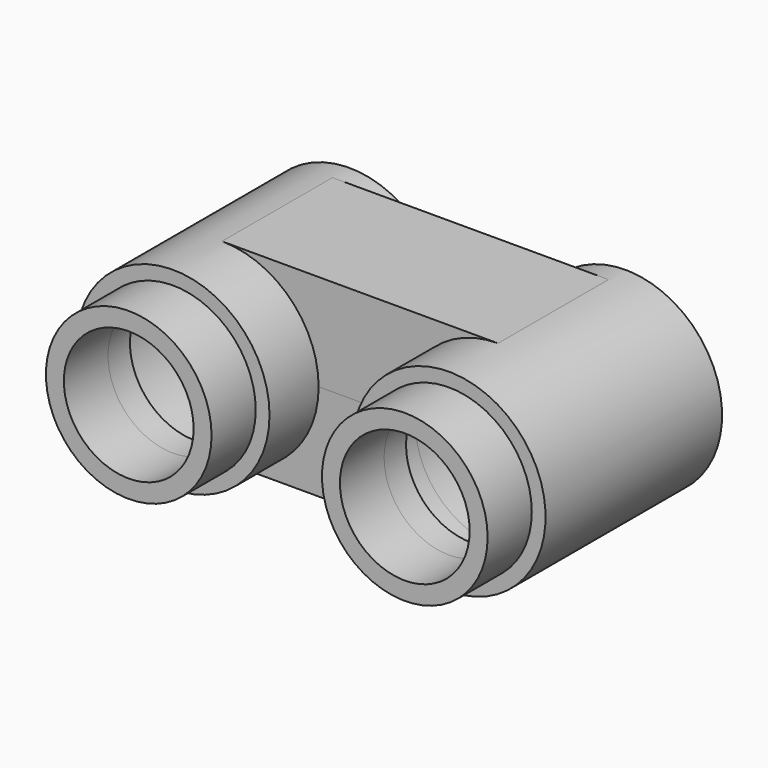
from build123d import *
from build123d import SkipClean  # not in build123d's __all__

# Parameters (mm, degrees)
F1_R           = 8.89
F1_R_2         = 5.969
F3_R           = 7.62
F3_R_2         = 5.969
F4_R           = 7.62
F4_R_2         = 5.969
F5_DEPTH       = 5.08
F6_DEPTH       = 25.4
F6_DEPTH_BACK  = 25.4
F7_R           = 7.62
F8_R           = 7.62
F9_DEPTH       = 17.78
F0_W           = 25.4
F0_H           = 12.7
F10_DEPTH      = 8.89
F10_DEPTH_BACK = 8.89
F11_DEPTH      = 17.78


# Not quite as in the source:
# - a feature of the source that left no trace in its solid (it failed there, or was rolled back) is left out


with BuildPart() as f2:
    # F2: sweep along a path in F0
    with BuildLine(Plane.XY) as f2_path:
        Line((0, 0), (0, 35.9156))
        ThreePointArc((0, 35.9156), (12.7, 48.6156), (25.4, 35.9156))
        Line((25.4, 35.9156), (25.4, 0))
    # F1 (on Front) → F2 (sweep)
    with BuildSketch(Plane.XZ):
        Circle(F1_R)
        Circle(F1_R_2, mode=Mode.SUBTRACT)
    sweep(path=f2_path.line)

    # F3 (on face) + F4 (on face) → F5 (join)
    with BuildSketch(Plane.XZ):
        Circle(F3_R)
        Circle(F3_R_2, mode=Mode.SUBTRACT)
    with BuildSketch(Plane.XZ):
        with Locations((25.4, 0)):
            Circle(F4_R)
        with Locations((25.4, 0)):
            Circle(F4_R_2, mode=Mode.SUBTRACT)
    with SkipClean():  # cleaning this boolean's faces spoils the solid; the shape is the same uncleaned
        extrude(amount=F5_DEPTH)

    # F0 (on Top) → F6 (cut, two sides)
    with BuildSketch(Plane.XY) as f6_sk:
        with BuildLine():
            Line((-12.2957220301, 20.301265642), (0, 20.301265642))
            Line((0, 20.301265642), (0, 35.9156))
            ThreePointArc((0, 35.9156), (3.7197438789, 44.8958561211), (12.7, 48.6156))
            ThreePointArc((12.7, 48.6156), (21.6802561211, 44.8958561211), (25.4, 35.9156))
            Line((25.4, 35.9156), (25.4, 20.301265642))
            Line((25.4, 20.301265642), (40.2239970863, 20.301265642))
            Line((40.2239970863, 20.301265642), (40.2239970863, 60.9702691436))
            Line((40.2239970863, 60.9702691436), (-12.2957220301, 60.9702691436))
            Line((-12.2957220301, 60.9702691436), (-12.2957220301, 20.301265642))
        make_face()
        with BuildLine():
            Line((0, 35.9156), (0, 20.301265642))
            Line((0, 20.301265642), (12.7, 20.301265642))
            Line((12.7, 20.301265642), (12.7, 48.6156))
            ThreePointArc((12.7, 48.6156), (3.7197438789, 44.8958561211), (0, 35.9156))
        make_face()
        with BuildLine():
            Line((12.7, 20.301265642), (25.4, 20.301265642))
            Line((25.4, 20.301265642), (25.4, 35.9156))
            ThreePointArc((25.4, 35.9156), (21.6802561211, 44.8958561211), (12.7, 48.6156))
            Line((12.7, 48.6156), (12.7, 20.301265642))
        make_face()
    extrude(amount=-F6_DEPTH, mode=Mode.SUBTRACT)
    extrude(f6_sk.sketch, amount=F6_DEPTH_BACK, mode=Mode.SUBTRACT)

    # F7 (on face) + F8 (on face) → F9 (cut)
    with BuildSketch(Plane(origin=(0, 20.301265642, 0), x_dir=(-1, 0, 0), z_dir=(0, 1, 0))):
        with Locations((-25.4, 0)):
            Circle(F7_R)
    with BuildSketch(Plane(origin=(0, 20.301265642, 0), x_dir=(-1, 0, 0), z_dir=(0, 1, 0))):
        Circle(F8_R)
    extrude(amount=-F9_DEPTH, mode=Mode.SUBTRACT)

    # F0 (on Top) → F10 (join, two sides)
    with BuildSketch(Plane.XY) as f10_sk:
        with Locations((12.7, 11.9974283338)):
            Rectangle(F0_W, F0_H)
    extrude(amount=F10_DEPTH)
    extrude(f10_sk.sketch, amount=-F10_DEPTH_BACK)

    # F7 (on face) + F8 (on face) → F11 (cut)
    with BuildSketch(Plane(origin=(0, 20.301265642, 0), x_dir=(-1, 0, 0), z_dir=(0, 1, 0))):
        with Locations((-25.4, 0)):
            Circle(F7_R)
    with BuildSketch(Plane(origin=(0, 20.301265642, 0), x_dir=(-1, 0, 0), z_dir=(0, 1, 0))):
        Circle(F8_R)
    extrude(amount=-F11_DEPTH, mode=Mode.SUBTRACT)


solid = f2.part
